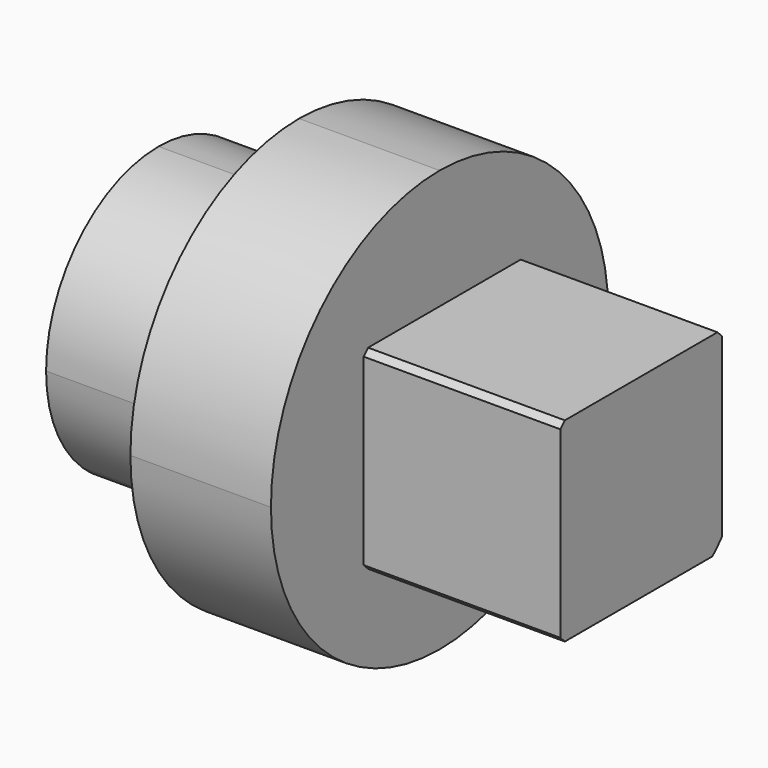
from build123d import *

# Parameters (mm, degrees)
F0_W          = 4.8315766917
F0_H          = 4.1204813641
F0_W_2        = 4.2928811043
F0_H_2        = 4.6790674097
F1_DEPTH      = 6.35
F1_DEPTH_BACK = 6.35
F2_DEPTH      = 6.35
F3_START      = 6.35
F3_DEPTH      = 8.89
F4_SIZE       = 0.254


# Not quite as in the source:
# - a feature names something its author has since deleted; it is built from what else it names


with BuildPart() as f1:
    # F0 (on Right) → F1 (new body, two sides)
    with BuildSketch(Plane.YZ) as f1_sk:
        with BuildLine():
            Line((0, -4.6790674097), (0, -6.35))
            ThreePointArc((0, -6.35), (1.9649498234, -6.0383335608), (3.7370149493, -5.1339282493))
            ThreePointArc((3.7370149493, -5.1339282493), (4.0213843703, -4.9143634121), (4.2928811043, -4.6790674097))
            Line((4.2928811043, -4.6790674097), (0, -4.6790674097))
        make_face()
        with BuildLine():
            Line((4.8315766917, -4.1204813641), (4.8315766917, 0))
            Line((4.8315766917, 0), (0, 0))
            Line((0, 0), (0, -4.6790674097))
            Line((0, -4.6790674097), (4.2928811043, -4.6790674097))
            ThreePointArc((4.2928811043, -4.6790674097), (4.5707698597, -4.4080112171), (4.8315766917, -4.1204813641))
        make_face()
        with Locations((2.4157883458, 2.0602406821)):
            Rectangle(F0_W, F0_H)
        with Locations((-2.1464405521, 2.0602406821)):
            Rectangle(F0_W_2, F0_H)
        with Locations((-2.1464405521, -2.3395337049)):
            Rectangle(F0_W_2, F0_H_2)
        with BuildLine():
            Line((-4.2928811043, 0), (-6.35, 0))
            ThreePointArc((-6.35, 0), (-5.813015354, -2.55565109), (-4.2928811043, -4.6790674097))
            Line((-4.2928811043, -4.6790674097), (-4.2928811043, 0))
        make_face()
        with BuildLine():
            ThreePointArc((-3.3540888173, -5.3919002407), (-1.7441234864, -6.105778678), (0, -6.35))
            Line((0, -6.35), (0, -4.6790674097))
            Line((0, -4.6790674097), (-4.2928811043, -4.6790674097))
            ThreePointArc((-4.2928811043, -4.6790674097), (-3.8400611852, -5.057314514), (-3.3540888173, -5.3919002407))
        make_face()
        with BuildLine():
            Line((4.8315766917, 0), (6.35, 0))
            ThreePointArc((6.35, 0), (5.958314023, 2.1956762065), (4.8315766917, 4.1204813641))
            Line((4.8315766917, 4.1204813641), (4.8315766917, 0))
        make_face()
        with BuildLine():
            ThreePointArc((4.8315766917, -4.1204813641), (5.958314023, -2.1956762065), (6.35, 0))
            Line((6.35, 0), (4.8315766917, 0))
            Line((4.8315766917, 0), (4.8315766917, -4.1204813641))
        make_face()
        with BuildLine():
            ThreePointArc((4.8315766917, 4.1204813641), (2.6605867151, 5.765741785), (0, 6.35))
            Line((0, 6.35), (0, 4.1204813641))
            Line((0, 4.1204813641), (4.8315766917, 4.1204813641))
        make_face()
        with BuildLine():
            Line((0, 4.1204813641), (0, 6.35))
            ThreePointArc((0, 6.35), (-4.4901280605, 4.4901280605), (-6.35, 0))
            Line((-6.35, 0), (-4.2928811043, 0))
            Line((-4.2928811043, 0), (-4.2928811043, 4.1204813641))
            Line((-4.2928811043, 4.1204813641), (0, 4.1204813641))
        make_face()
    extrude(amount=F1_DEPTH)
    extrude(f1_sk.sketch, amount=-F1_DEPTH_BACK)

    # F0 (on Right) → F2 (join)
    with BuildSketch(Plane.YZ):
        with BuildLine():
            ThreePointArc((0, -9.525), (6.7351920908, -6.7351920908), (9.525, 0))
            Line((9.525, 0), (6.35, 0))
            ThreePointArc((6.35, 0), (5.958314023, -2.1956762065), (4.8315766917, -4.1204813641))
            Line((4.8315766917, -4.1204813641), (4.8315766917, -4.6790674097))
            Line((4.8315766917, -4.6790674097), (4.2928811043, -4.6790674097))
            ThreePointArc((4.2928811043, -4.6790674097), (4.0213843703, -4.9143634121), (3.7370149493, -5.1339282493))
            ThreePointArc((3.7370149493, -5.1339282493), (1.9649498234, -6.0383335608), (0, -6.35))
            Line((0, -6.35), (0, -9.525))
        make_face()
        with BuildLine():
            Line((6.35, 0), (9.525, 0))
            ThreePointArc((9.525, 0), (6.7351920908, 6.7351920908), (0, 9.525))
            Line((0, 9.525), (0, 6.35))
            ThreePointArc((0, 6.35), (2.6605867151, 5.765741785), (4.8315766917, 4.1204813641))
            ThreePointArc((4.8315766917, 4.1204813641), (5.958314023, 2.1956762065), (6.35, 0))
        make_face()
        with BuildLine():
            Line((0, 6.35), (0, 9.525))
            ThreePointArc((0, 9.525), (-6.7351920908, 6.7351920908), (-9.525, 0))
            Line((-9.525, 0), (-6.35, 0))
            ThreePointArc((-6.35, 0), (-4.4901280605, 4.4901280605), (0, 6.35))
        make_face()
        with BuildLine():
            ThreePointArc((-9.525, 0), (-6.7351920908, -6.7351920908), (0, -9.525))
            Line((0, -9.525), (0, -6.35))
            ThreePointArc((0, -6.35), (-1.7441234864, -6.105778678), (-3.3540888173, -5.3919002407))
            ThreePointArc((-3.3540888173, -5.3919002407), (-3.8400611852, -5.057314514), (-4.2928811043, -4.6790674097))
            ThreePointArc((-4.2928811043, -4.6790674097), (-5.813015354, -2.55565109), (-6.35, 0))
            Line((-6.35, 0), (-9.525, 0))
        make_face()
    extrude(amount=F2_DEPTH)

    # F0 (on Right) → F3 (join)
    with BuildSketch(Plane.YZ.offset(F3_START)):
        with BuildLine():
            Line((4.8315766917, -4.1204813641), (4.8315766917, 0))
            Line((4.8315766917, 0), (0, 0))
            Line((0, 0), (0, -4.6790674097))
            Line((0, -4.6790674097), (4.2928811043, -4.6790674097))
            ThreePointArc((4.2928811043, -4.6790674097), (4.5707698597, -4.4080112171), (4.8315766917, -4.1204813641))
        make_face()
        with Locations((2.4157883458, 2.0602406821)):
            Rectangle(F0_W, F0_H)
        with Locations((-2.1464405521, 2.0602406821)):
            Rectangle(F0_W_2, F0_H)
        with Locations((-2.1464405521, -2.3395337049)):
            Rectangle(F0_W_2, F0_H_2)
    extrude(amount=F3_DEPTH)

    # F4
    f4_edges = [f1.edges().sort_by_distance(p)[0] for p in [
        (10.795, -4.292881, 4.120481),
        (10.795, -4.292881, -4.679067),
        (10.795, 4.831577, 4.120481),
    ]]
    chamfer(f4_edges, length=F4_SIZE)


solid = f1.part
